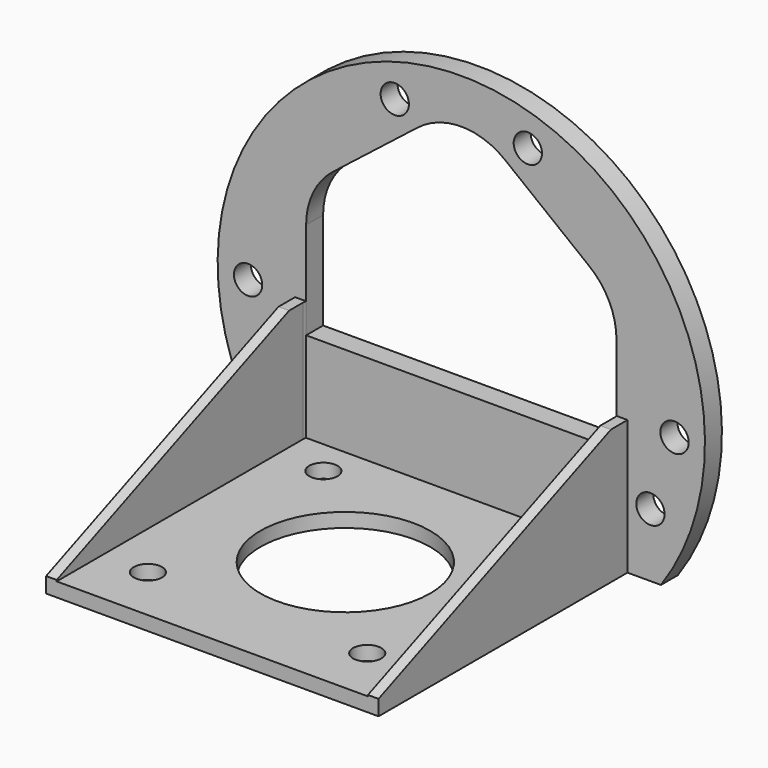
from build123d import *

# Parameters (mm, degrees)
F1_DEPTH         = 19
F0_W             = 44.0000004768
F0_H             = 45.5000002384
F0_R             = 12
F2_DEPTH         = 2
F3_D             = 4
F5_DEPTH         = 50
F7_DEPTH         = 3
F8_D             = 4
F9_R             = 2
F10_R            = 34.4476203659
F10_W            = 47
F10_H            = 19
F6_W             = 47
F6_H             = 19
F11_DEPTH        = 3
F13_DEPTH        = 25
F14_D            = 4
F14_DEPTH        = 6
F14_TIP          = 1.2017212381
F14_ON_F12_D     = 4
F14_ON_F12_DEPTH = 6
F14_ON_F12_TIP   = 1.2017212381


# Not quite as in the source:
# - a feature names something its author has since deleted; it is built from what else it names


with BuildPart() as f1:
    # F0 (on Top) → F1 (new body)
    with BuildSketch(Plane.XY):
        Polygon((23.5, -23.5), (23.5, 23.5), (-23.5, 23.5), (-23.5, -23.5), (-22.0000002384, -23.5), (-22.0000002384, 22.0000002384), (22.0000002384, 22.0000002384), (22.0000002384, -23.5), align=None)
    extrude(amount=F1_DEPTH)

    # F0 (on Top) → F2 (join)
    with BuildSketch(Plane.XY):
        with Locations((0, -0.7499998808)):
            Rectangle(F0_W, F0_H)
        Circle(F0_R, mode=Mode.SUBTRACT)
    extrude(amount=F2_DEPTH)

    # F3 (through all)
    with Locations(Plane(origin=(0, 0, 0), x_dir=(1, 0, 0), z_dir=(0, 0, -1))):
        with Locations((-15.5, -15.5), (15.5, -15.5), (15.5, 15.5), (-15.5, 15.5)):
            Hole(F3_D / 2)

    # F4 (on face) → F5 (cut)
    with BuildSketch(Plane.YZ.offset(23.5)):
        Polygon((-23.5, 19), (-23.5, 2.1775800269), (17.5668895245, 19), align=None)
    extrude(amount=-F5_DEPTH, mode=Mode.SUBTRACT)

    # F6 (on face) → F7 (join)
    with BuildSketch(Plane(origin=(0, 23.5, 0), x_dir=(-1, 0, 0), z_dir=(0, 1, 0))):
        with BuildLine():
            Line((-23.5, 19), (-25.1444590574, 19))
            ThreePointArc((-25.1444590574, 19), (-28.6799929633, 17.5355339059), (-30.1444590574, 14))
            Line((-30.1444590574, 14), (-30.1444590574, 5))
            ThreePointArc((-30.1444590574, 5), (-28.6799929633, 1.4644660941), (-25.1444590574, 0))
            Line((-25.1444590574, 0), (-23.5, 0))
            Line((-23.5, 0), (-23.5, 19))
        make_face()
        with BuildLine():
            Line((24.0855421871, 19), (23.5, 19))
            Line((23.5, 19), (23.5, 0))
            Line((23.5, 0), (24.0855421871, 0))
            ThreePointArc((24.0855421871, 0), (27.621076093, 1.4644660941), (29.0855421871, 5))
            Line((29.0855421871, 5), (29.0855421871, 14))
            ThreePointArc((29.0855421871, 14), (27.621076093, 17.5355339059), (24.0855421871, 19))
        make_face()
    extrude(amount=-F7_DEPTH)

    # F8 (through all)
    with Locations(Plane(origin=(0, 23.5, 0), x_dir=(-1, 0, 0), z_dir=(0, 1, 0))):
        with Locations((-26.7366040498, 8.9737372473), (28.2633959502, 9.5)):
            Hole(F8_D / 2)

    # F9
    f9_edges = [f1.edges().sort_by_distance(p)[0] for p in [
        (22, 22, 10.5),
        (-22, 22, 10.5),
    ]]
    fillet(f9_edges, radius=F9_R)

    # F10 (on face) + F6 (on face) → F11 (join)
    with BuildSketch(Plane(origin=(0, 23.5, 0), x_dir=(-1, 0, 0), z_dir=(0, 1, 0))):
        with Locations((0, 19.7549201548)):
            Circle(F10_R)
        with Locations((0, 9.5)):
            Rectangle(F10_W, F10_H, mode=Mode.SUBTRACT)
    with BuildSketch(Plane(origin=(0, 23.5, 0), x_dir=(-1, 0, 0), z_dir=(0, 1, 0))):
        with Locations((0, 9.5)):
            Rectangle(F6_W, F6_H)
    extrude(amount=-F11_DEPTH)

    # F12 (on face) → F13 (cut)
    with BuildSketch(Plane(origin=(0, 23.5, 0), x_dir=(-1, 0, 0), z_dir=(0, 1, 0))):
        with BuildLine():
            ThreePointArc((-18.1099253817, 36.3759554919), (-20.9291093364, 32.8831264718), (-21.9364919731, 28.5090170817))
            Line((-21.9364919731, 28.5090170817), (-21.9364919731, 14.7631261498))
            Line((-21.9364919731, 14.7631261498), (21.9364919731, 14.7631261498))
            Line((21.9364919731, 14.7631261498), (21.9364919731, 28.5090170817))
            ThreePointArc((21.9364919731, 28.5090170817), (20.9291093364, 32.8831264718), (18.1099253817, 36.3759554919))
            Line((18.1099253817, 36.3759554919), (6.1734334086, 45.7428952702))
            ThreePointArc((6.1734334086, 45.7428952702), (0, 47.87595686), (-6.1734334086, 45.7428952702))
            Line((-6.1734334086, 45.7428952702), (-18.1099253817, 36.3759554919))
        make_face()
        with BuildLine():
            Line((28.2202352675, 0), (-28.2202352675, 0))
            ThreePointArc((-28.2202352675, 0), (0, -14.6927002111), (28.2202352675, 0))
        make_face()
    extrude(amount=-F13_DEPTH, mode=Mode.SUBTRACT)

    # F14
    with Locations(Plane(origin=(0, 23.5, 0), x_dir=(-1, 0, 0), z_dir=(0, 1, 0))):
        with Locations((-30.1444590574, 19), (-26.7366040498, 8.9737372473), (26.7366040498, 8.9737372473), (30.1444590574, 19)):
            Hole(F14_D / 2, depth=F14_DEPTH)
            with Locations((0, 0, -(F14_DEPTH + F14_TIP / 2))):  # 118° drill point
                Cone(0, F14_D / 2, F14_TIP, mode=Mode.SUBTRACT)

    # F14 on F12
    with Locations(Plane(origin=(0, 23.5, 0), x_dir=(-1, 0, 0), z_dir=(0, 1, 0))):
        with Locations((9.4067957252, 48.2378602028), (-9.4067957252, 48.2378602028)):
            Hole(F14_ON_F12_D / 2, depth=F14_ON_F12_DEPTH)
            with Locations((0, 0, -(F14_ON_F12_DEPTH + F14_ON_F12_TIP / 2))):  # 118° drill point
                Cone(0, F14_ON_F12_D / 2, F14_ON_F12_TIP, mode=Mode.SUBTRACT)


solid = f1.part
